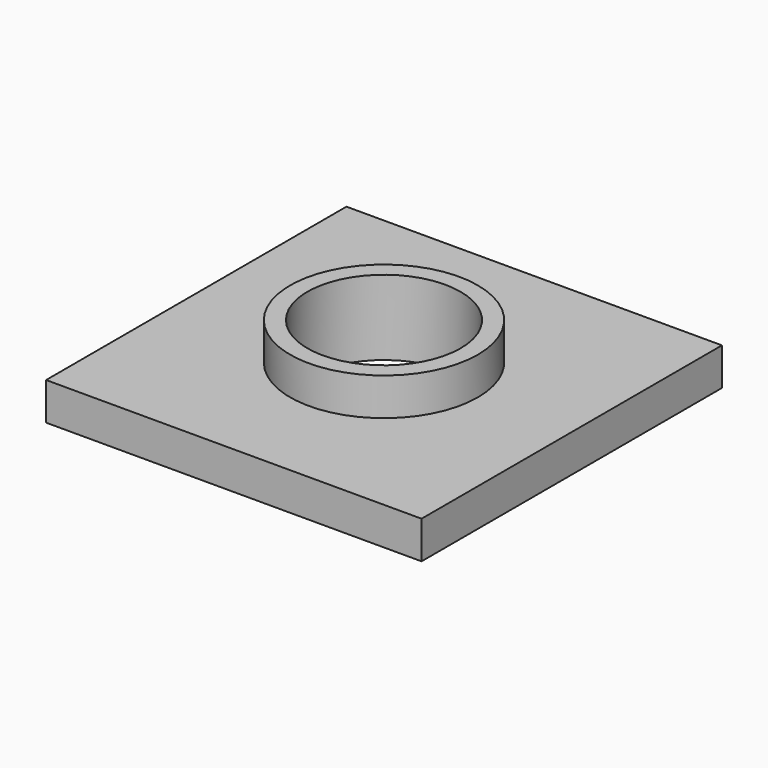
from build123d import *

# Parameters (mm, degrees)
F0_R     = 2.5
F0_R_2   = 2.04
F1_DEPTH = 1
F2_R     = 2.5
F2_R_2   = 2.04
F3_DEPTH = 1


with BuildPart() as f1:
    # F0 (on Top) → F1 (new body)
    with BuildSketch(Plane.XY):
        Circle(F0_R)
        Circle(F0_R_2, mode=Mode.SUBTRACT)
    extrude(amount=F1_DEPTH)

    # F2 (on face) → F3 (join)
    with BuildSketch(Plane(origin=(0, 0, 0), x_dir=(1, 0, 0), z_dir=(0, 0, -1))):
        with BuildLine():
            ThreePointArc((0, -5), (3.5355339059, -3.5355339059), (5, 0))
            ThreePointArc((5, 0), (3.5355339059, 3.5355339059), (0, 5))
            ThreePointArc((0, 5), (-3.5355339059, 3.5355339059), (-5, 0))
            ThreePointArc((-5, 0), (-3.5355339059, -3.5355339059), (0, -5))
        make_face()
        Circle(F2_R, mode=Mode.SUBTRACT)
        with BuildLine():
            Line((5, -5), (5, 0))
            ThreePointArc((5, 0), (3.5355339059, -3.5355339059), (0, -5))
            Line((0, -5), (5, -5))
        make_face()
        with BuildLine():
            ThreePointArc((0, 5), (3.5355339059, 3.5355339059), (5, 0))
            Line((5, 0), (5, 5))
            Line((5, 5), (0, 5))
        make_face()
        with BuildLine():
            ThreePointArc((-5, 0), (-3.5355339059, 3.5355339059), (0, 5))
            Line((0, 5), (-5, 5))
            Line((-5, 5), (-5, 0))
        make_face()
        with BuildLine():
            Line((-5, -5), (0, -5))
            ThreePointArc((0, -5), (-3.5355339059, -3.5355339059), (-5, 0))
            Line((-5, 0), (-5, -5))
        make_face()
        Circle(F2_R)
        Circle(F2_R_2, mode=Mode.SUBTRACT)
    extrude(amount=F3_DEPTH)


solid = f1.part
